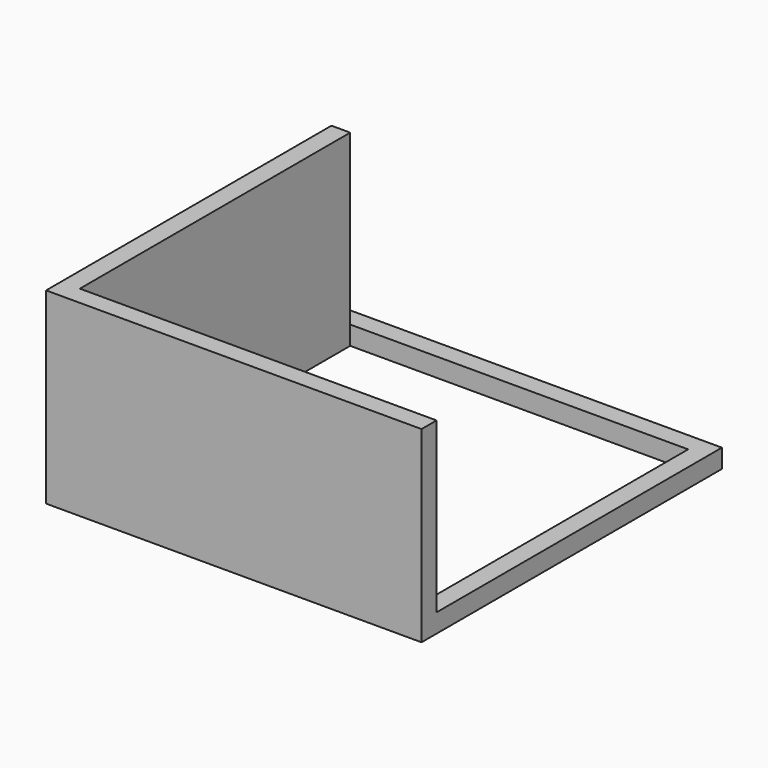
from build123d import *

# Parameters (mm, degrees)
F0_W     = 50
F0_H     = 50
F1_DEPTH = 25
F2_T     = -2.5
F3_T     = 2.5


# Not quite as in the source:
# - a shell that OpenCascade refuses in one call is made with other operations: the cavity is built on its own and cut out


with BuildPart() as f1:
    # F0 (on Top) → F1 (new body)
    with BuildSketch(Plane.XY):
        with Locations((0.357497856, 6.2575038522)):
            Rectangle(F0_W, F0_H)
    extrude(amount=F1_DEPTH)

    # F2
    f2_openings = [f1.faces().sort_by_distance(p)[0] for p in [
        (0.357498, 6.257504, 25),
        (0.357498, 6.257504, 0),
    ]]
    offset(amount=F2_T, openings=f2_openings)

    # F3: shell of thickness 2.5, made by hand


with BuildPart() as f3_core1:
    # F3_t2: copy of F1
    add(f1.part)

    # the walls: a layer under each face that stays
    f3_faces = [f3_core1.faces().sort_by_distance(p)[0] for p in [
        (0.357497856, -18.7424961478, 12.5),
        (-22.9758354773, -17.0758294811, 0),
        (-22.142502144, 6.2575038522, 12.5),
    ]]
    thicken(f3_faces, amount=-F3_T, mode=Mode.SUBTRACT)


with BuildPart() as f1_1:
    add(f1.part)

    # what is left inside the walls is the cavity
    f3_cavity = [f3_core1.part.solids().sort_by_distance(p)[0] for p in [
        (0.357498, 31.232504, 17.5),
    ]]
    add(f3_cavity, mode=Mode.SUBTRACT)


solid = f1_1.part
